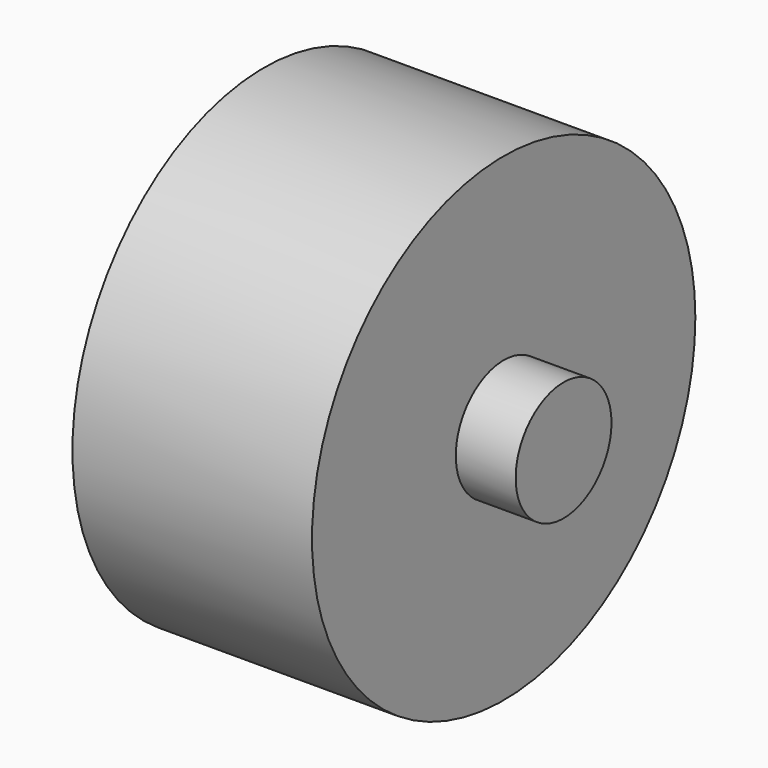
from build123d import *

# Parameters (mm, degrees)
F0_R     = 3.175
F1_DEPTH = 9.525
F0_R_2   = 12.7
F2_DEPTH = 6.35


# Not quite as in the source:
# - a feature of the source that left no trace in its solid (it failed there, or was rolled back) is left out


with BuildPart() as f1:
    # F0 (on Right) → F1 (new body, symmetric)
    with BuildSketch(Plane.YZ):
        Circle(F0_R)
    extrude(amount=F1_DEPTH, both=True)

    # F0 (on Right) → F2 (join, symmetric)
    with BuildSketch(Plane.YZ):
        Circle(F0_R_2)
        Circle(F0_R, mode=Mode.SUBTRACT)
    extrude(amount=F2_DEPTH, both=True)


solid = f1.part
